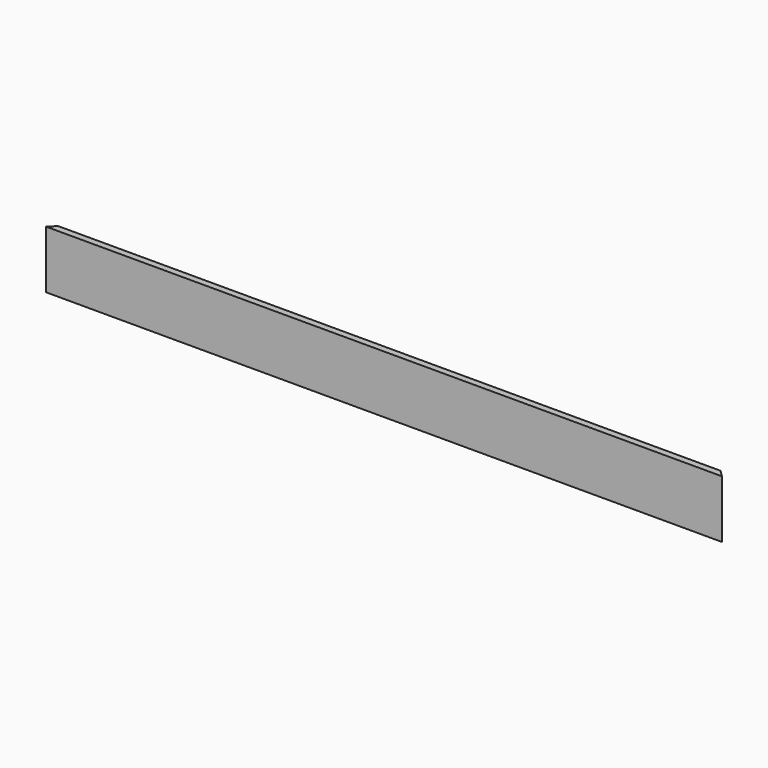
from build123d import *

# Parameters (mm, degrees)
F0_W     = 1930.4
F0_H     = 165.1
F1_DEPTH = 19.05
F2_SIZE  = 19.04999


# Not quite as in the source:
# - a fillet or chamfer is up to 0.001 mm smaller than in the source, because OpenCascade refuses the exact size


with BuildPart() as f1:
    # F0 (on Front) → F1 (new body)
    with BuildSketch(Plane.XZ):
        Rectangle(F0_W, F0_H)
    extrude(amount=F1_DEPTH)

    # F2 (size 19.05 in the source; OpenCascade refuses exactly that, so slightly less here)
    f2_edges = [f1.edges().sort_by_distance(p)[0] for p in [
        (965.2, 0, 0),
        (-965.2, 0, 0),
    ]]
    chamfer(f2_edges, length=F2_SIZE)


solid = f1.part
